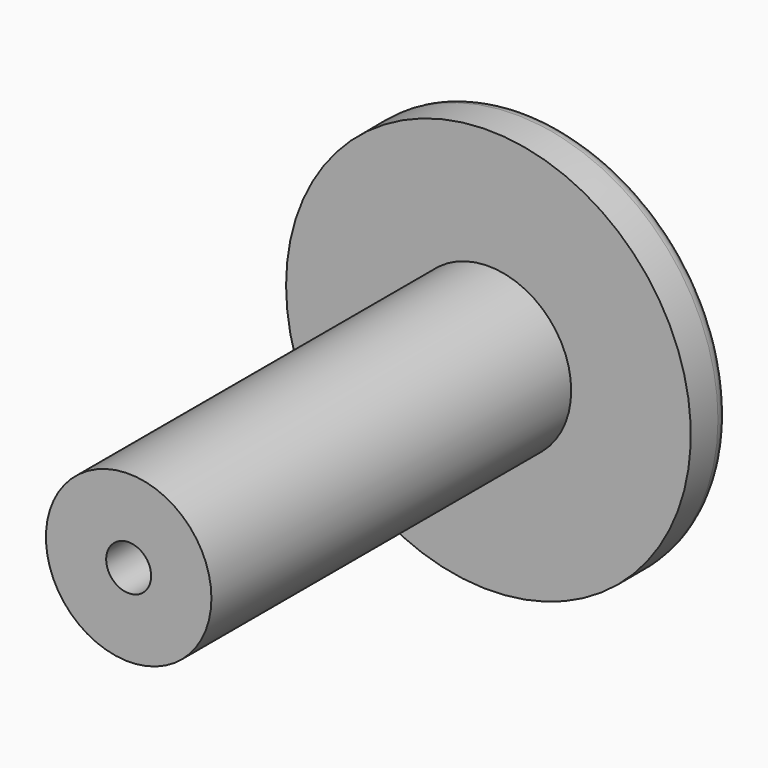
from build123d import *

# Parameters (mm, degrees)
F0_R     = 2.921
F1_DEPTH = 19.05
F2_R     = 7.14375
F2_R_2   = 2.921
F3_DEPTH = 3.175
F4_R     = 0.79375
F5_DEPTH = 19.051
F8_R     = 0.508


# Not quite as in the source:
# - a feature names something its author has since deleted; it is built from what else it names


with BuildPart() as f1:
    # F0 (on Front) → F1 (new body)
    with BuildSketch(Plane.XZ):
        Circle(F0_R)
    extrude(amount=-F1_DEPTH)

    # F2 (on face) → F3 (join)
    with BuildSketch(Plane(origin=(0, 19.05, 0), x_dir=(-1, 0, 0), z_dir=(0, 1, 0))):
        Circle(F2_R)
        Circle(F2_R_2, mode=Mode.SUBTRACT)
    extrude(amount=-F3_DEPTH)

    # F4 (on face) → F5 (cut, through all)
    with BuildSketch(Plane.XZ):
        Circle(F4_R)
    extrude(amount=-F5_DEPTH, mode=Mode.SUBTRACT)

    # F6 (on Right) → F7 (revolve, cut)
    with BuildSketch(Plane.YZ):
        with BuildLine():
            ThreePointArc((19.0884582698, 0), (18.6124325104, -3.7323455074), (17.335280776, -7.2715384886))
            Line((17.335280776, -7.2715384886), (21.6284582698, -7.2715384886))
            Line((21.6284582698, -7.2715384886), (21.6284582698, 0))
            Line((21.6284582698, 0), (19.0884582698, 0))
        make_face()
    revolve(axis=Axis((0, 12.9899214953, 0), (0, 1, 0)), mode=Mode.SUBTRACT)

    # F8
    f8_edges = [f1.edges().sort_by_distance(p)[0] for p in [
        (5.051394, 17.397311, 5.051394),
        (-5.051394, 17.397311, -5.051394),
    ]]
    fillet(f8_edges, radius=F8_R)


solid = f1.part
